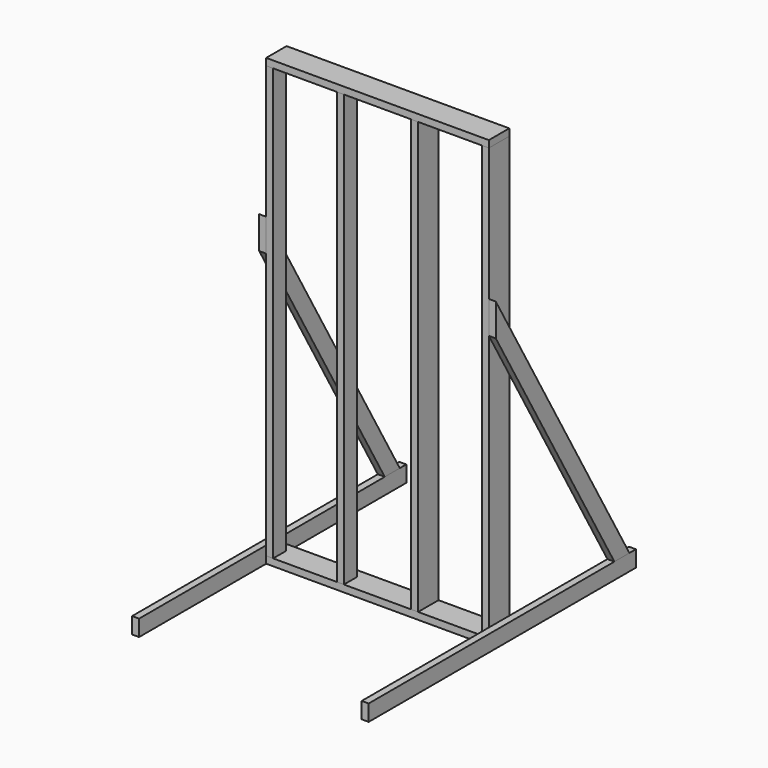
from build123d import *

# Parameters (mm, degrees)
F0_W          = 38.1
F0_H          = 2362.2
F1_DEPTH      = 88.9
F3_W          = 1219.2
F3_H          = 38.1
F4_DEPTH      = 88.9
F4_DEPTH_BACK = 50.8
F6_W          = 1828.8
F6_H          = 88.9
F7_DEPTH      = 38.1
F10_W         = 139.7
F10_H         = 2362.2
F11_DEPTH     = 38.1
F14_DEPTH     = 38.1


# Not quite as in the source:
# - a feature of the source that left no trace in its solid (it failed there, or was rolled back) is left out
# - a pattern or mirror of a feature is missing from the dataset's text; its kind, count and spacing are read off the source's solid


with BuildPart() as f1:
    # F0 (on Front) → F1 (new body)
    with BuildSketch(Plane.XZ):
        with Locations((19.05, 1181.1)):
            Rectangle(F0_W, F0_H)
    extrude(amount=F1_DEPTH)


with BuildPart() as f2_1:
    # F2: copy of F1
    add(f1.part.moved(Location((387.35, 0, 0))))


with BuildPart() as f4:
    # F3 (on Front) → F4 (new body, two sides)
    with BuildSketch(Plane.XZ) as f4_sk:
        with Locations((609.6, -19.05)):
            Rectangle(F3_W, F3_H)
    extrude(amount=F4_DEPTH)
    extrude(f4_sk.sketch, amount=-F4_DEPTH_BACK)


with BuildPart() as f4_copies_1:
    # F4_copies: instance of F4
    add(f4.part.mirror(Plane.XY.offset(1181.1)))


with BuildPart() as f7:
    # F6 (on face) → F7 (new body)
    with BuildSketch(Plane(origin=(0, 0, 0), x_dir=(0, -1, 0), z_dir=(-1, 0, 0))):
        with Locations((44.45, 6.35)):
            Rectangle(F6_W, F6_H)
    extrude(amount=F7_DEPTH)


with BuildPart() as f8_1:
    # F8: copy of F7
    add(f7.part.moved(Location((1257.3, 0, 0))))


with BuildPart() as f11:
    # F10 (on offset) → F11 (new body)
    with BuildSketch(Plane.YZ.offset(793.75)):
        with Locations((-19.05, 1181.1)):
            Rectangle(F10_W, F10_H)
    extrude(amount=F11_DEPTH)


with BuildPart() as f12_1:
    # F12: copy of F11
    add(f11.part.moved(Location((387.35, 0, 0))))


with BuildPart() as f14:
    # F13 (on face) → F14 (new body)
    with BuildSketch(Plane(origin=(1219.2, 0, 0), x_dir=(0, -1, 0), z_dir=(-1, 0, 0))):
        Polygon((0, 1480.6079416481), (-825.5, 50.8), (-722.8471221381, 50.8), (0, 1302.8079416481), align=None)
        Polygon((88.9, 1634.587258441), (0, 1480.6079416481), (0, 1302.8079416481), (88.9, 1456.787258441), align=None)
    extrude(amount=-F14_DEPTH)


with BuildPart() as f15_1:
    # F15: copy of F14
    add(f14.part.moved(Location((-1257.3, 0, 0))))


solid = Compound([f1.part, f2_1.part, f4.part, f4_copies_1.part, f7.part, f8_1.part, f11.part, f12_1.part, f14.part, f15_1.part])
